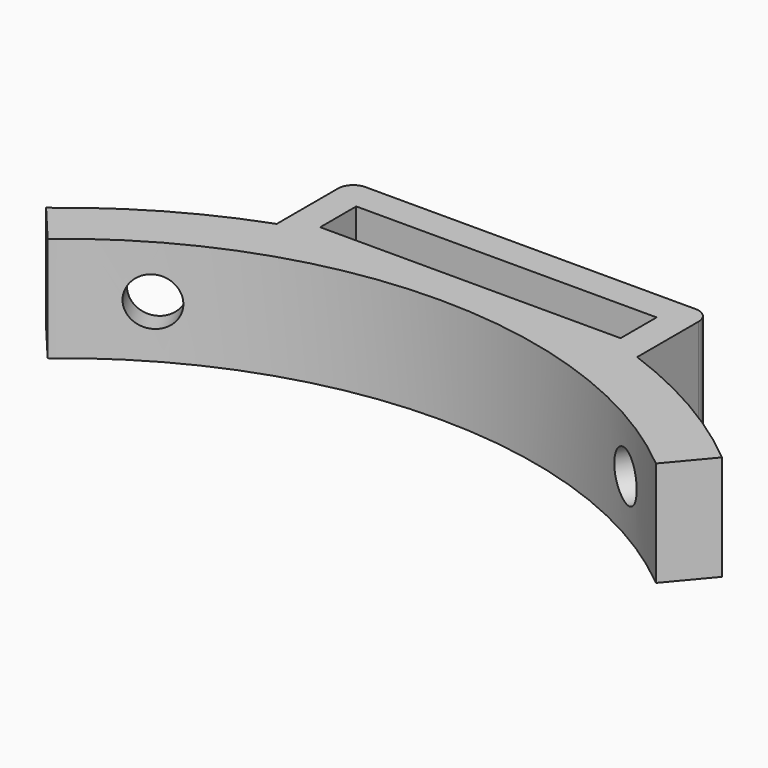
from build123d import *

# Parameters (mm, degrees)
F0_R      = 35
F0_R_2    = 31.5
F1_DEPTH  = 3.5
F2_W      = 20
F2_H      = 3
F3_DEPTH  = 3.5
F4_DEPTH  = 12.5
F9_W      = 10.4753747582
F9_H      = 9.4332345761
F10_ANGLE = 280


# Not quite as in the source:
# - a feature names something its author has since deleted; it is built from what else it names


with BuildPart() as f1:
    # F0 (on Top) → F1 (new body, symmetric)
    with BuildSketch(Plane.XY):
        Circle(F0_R)
        Circle(F0_R_2, mode=Mode.SUBTRACT)
    extrude(amount=F1_DEPTH, both=True)

    # F2 (on Top) → F3 (join, symmetric)
    with BuildSketch(Plane.XY):
        with BuildLine():
            ThreePointArc((12, 38), (11.7071067812, 38.7071067812), (11, 39))
            Line((11, 39), (-11, 39))
            ThreePointArc((-11, 39), (-11.7071067812, 38.7071067812), (-12, 38))
            Line((-12, 38), (-12, 31.5))
            Line((-12, 31.5), (12, 31.5))
            Line((12, 31.5), (12, 38))
        make_face()
        with Locations((0, 35.5)):
            Rectangle(F2_W, F2_H, mode=Mode.SUBTRACT)
    extrude(amount=F3_DEPTH, both=True)

    # F2 (on Top) → F4 (cut, symmetric)
    with BuildSketch(Plane.XY):
        with Locations((0, 35.5)):
            Rectangle(F2_W, F2_H)
    extrude(amount=F4_DEPTH, both=True, mode=Mode.SUBTRACT)

    # F9 (on face) → F10 (revolve, cut)
    with BuildSketch(Plane(origin=(0, 0, 0), x_dir=(0.6427876097, 0.7660444431, 0), z_dir=(0.7660444431, -0.6427876097, 0))):
        with Locations((33.1802591681, -0.398933189)):
            Rectangle(F9_W, F9_H)
    revolve(axis=Axis((0, 0, 0), (0, 0, -1)), revolution_arc=F10_ANGLE, mode=Mode.SUBTRACT)

    # F5 (on Top) → F11 (revolve, cut)
    with BuildSketch(Plane.XY):
        Polygon((16.5, 28.5788383249), (17.8856406461, 27.7788383249), (19.0980762114, 27.0788383249), (20.7630293139, 29.9626216907), (18.1649531025, 31.4626216907), align=None)
        Polygon((16.0922047839, 24.6725162916), (17.8856406461, 27.7788383249), (16.5, 28.5788383249), (14.7065641379, 25.4725162916), align=None)
    revolve(axis=Axis((15.0315794057, 26.0354592487, 0), (0.5, 0.8660254038, 0)), mode=Mode.SUBTRACT)

    # F6 (on Top) → F12 (revolve, cut)
    with BuildSketch(Plane.XY):
        Polygon((-19.0980762114, 27.0788383249), (-17.8856406461, 27.7788383249), (-16.5, 28.5788383249), (-17.8281544713, 30.8792693496), (-20.4262306827, 29.3792693496), align=None)
        Polygon((-16.5, 28.5788383249), (-17.8856406461, 27.7788383249), (-16.1036535179, 24.6923460805), (-14.7180128719, 25.4923460805), align=None)
    revolve(axis=Axis((-13.6687379183, 23.6749485498, 0), (-0.5, 0.8660254038, 0)), mode=Mode.SUBTRACT)


solid = f1.part
